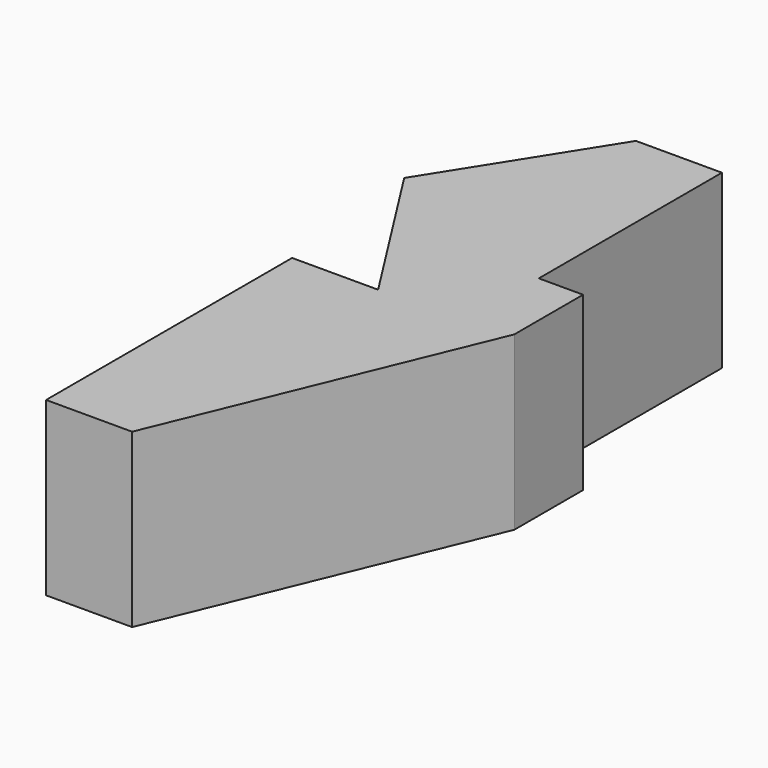
from build123d import *

# Parameters (mm, degrees)
F1_DEPTH = 25.4
F2_DEPTH = 25.4
F3_DEPTH = 25.4
F4_DEPTH = 25.4
F5_DEPTH = 25.4


with BuildPart() as f1:
    # F0 (on Top) → F1 (new body)
    with BuildSketch(Plane.XY):
        Polygon((29.9969874322, 40.0068945546), (29.9969874322, 6.1151932525), (51.8570691347, 5.7021006942), align=None)
        Polygon((51.8570691347, 5.7021006942), (29.9969874322, 6.1151932525), (29.9969874322, -50.8127212524), (68.4659332037, 42.1804785728), (29.9969874322, 42.1804785728), (29.9969874322, 40.0068945546), align=None)
        Polygon((-0.1684613526, 87.345212698), (29.9969874322, 40.0068945546), (29.9969874322, 42.1804785728), (29.9969874322, 135.1736783981), align=None)
    extrude(amount=F1_DEPTH)

    # F2 (add): a face of the model
    f2_faces = [f1.faces().sort_by_distance(p)[0] for p in [
        (29.9969874322, 88.6770784855, 12.7),
    ]]
    extrude(f2_faces, amount=F2_DEPTH)

    # F3 (add): a face of the model
    f3_faces = [f1.faces().sort_by_distance(p)[0] for p in [
        (36.8893007779, 63.5629589231, 0),
    ]]
    extrude(f3_faces, amount=F3_DEPTH)

    # F4 (add): a face of the model
    f4_faces = [f1.faces().sort_by_distance(p)[0] for p in [
        (61.931460318, 42.1804785728, 0),
    ]]
    extrude(f4_faces, amount=F4_DEPTH)

    # F5 (add): a face of the model
    f5_faces = [f1.faces().sort_by_distance(p)[0] for p in [
        (29.9969874322, -5.4029133489, 0),
    ]]
    extrude(f5_faces, amount=F5_DEPTH)


solid = f1.part
